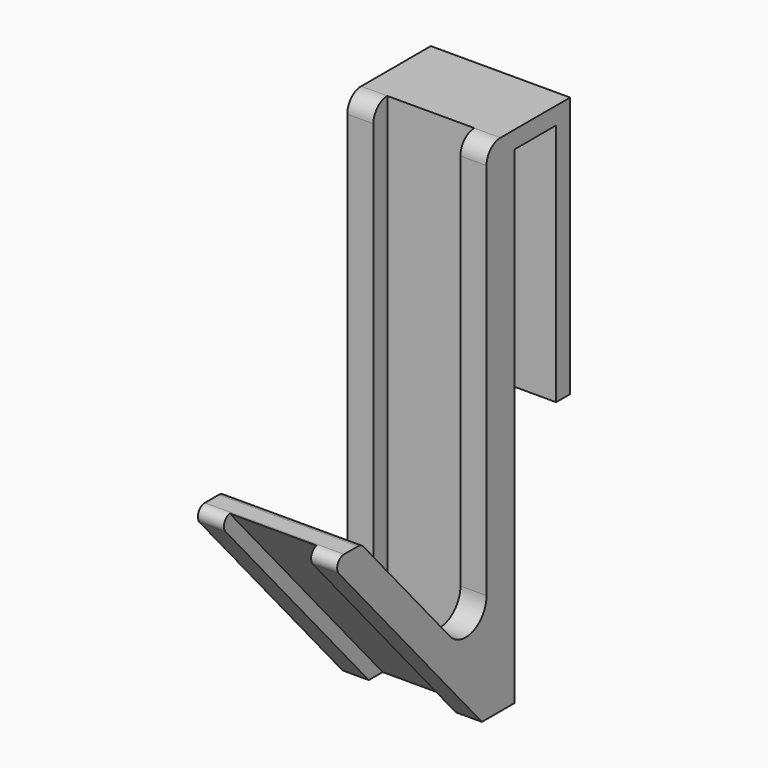
from build123d import *

# Parameters (mm, degrees)
F1_DEPTH = 16
F2_W     = 3
F2_H     = 2
F3_DEPTH = 58
F4_W     = 10
F4_H     = 2
F6_F1_R  = 0.9999
F7_R     = 1
F8_R     = 2
F9_R     = 3


# Not quite as in the source:
# - a fillet or chamfer is up to 0.001 mm smaller than in the source, because OpenCascade refuses the exact size


with BuildPart() as f1:
    # F0 (on Right) → F1 (new body)
    with BuildSketch(Plane.YZ):
        Polygon((-61.7935170661, -87.8824494406), (-61.7935170661, -143.6097221679), (-81.7935170661, -120.8824494406), (-86.4557482916, -120.8824494406), (-64.4557482916, -145.8824494406), (-59.7935170661, -145.8824494406), (-59.7935170661, -89.8824494406), (-53.7935170661, -89.8824494406), (-53.7935170661, -117.8824494406), (-51.7935170661, -117.8824494406), (-51.7935170661, -87.8824494406), align=None)
    extrude(amount=F1_DEPTH)

    # F2 (on face) → F3 (join)
    with BuildSketch(Plane.XY.offset(-87.8824494406)):
        with Locations((1.5, -62.7935170661)):
            Rectangle(F2_W, F2_H)
        with Locations((14.5, -62.7935170661)):
            Rectangle(F2_W, F2_H)
    extrude(amount=-F3_DEPTH)

    # F5: sweep along a path in F5_path
    with BuildLine(Plane(origin=(16, -64.4557482916, -145.8824494406), x_dir=(0, 0.6606278949, -0.7507135169), z_dir=(0, 0.7507135169, 0.6606278949))) as f5_path:
        Line((0, 0), (-33.3016516107, 0))
    # F4 (on face) → F5 (sweep, cut)
    with BuildSketch(Plane.XY.offset(-120.8824494406)):
        with Locations((8, -85.4557482916)):
            Rectangle(F4_W, F4_H)
    sweep(path=f5_path.line, mode=Mode.SUBTRACT)

    # F6: fillet of radius 1 on 2 edges, made by hand

    # F6_f1 (radius 1 in the source; OpenCascade refuses exactly that, so slightly less here)
    f6_f1_edges = [f1.edges().sort_by_distance(p)[0] for p in [
        (1.5, -86.4557482916, -120.8824494406),
    ]]
    fillet(f6_f1_edges, radius=F6_F1_R)

    # F7
    f7_edges = [f1.edges().sort_by_distance(p)[0] for p in [
        (8, -81.793517, -120.882449),
    ]]
    fillet(f7_edges, radius=F7_R)

    # F8
    f8_edges = [f1.edges().sort_by_distance(p)[0] for p in [
        (14.5, -63.793517, -87.882449),
        (1.5, -63.793517, -87.882449),
    ]]
    fillet(f8_edges, radius=F8_R)

    # F9
    f9_edges = [f1.edges().sort_by_distance(p)[0] for p in [
        (14.5, -63.793517, -141.336995),
        (1.5, -63.793517, -141.336995),
    ]]
    fillet(f9_edges, radius=F9_R)


solid = f1.part
